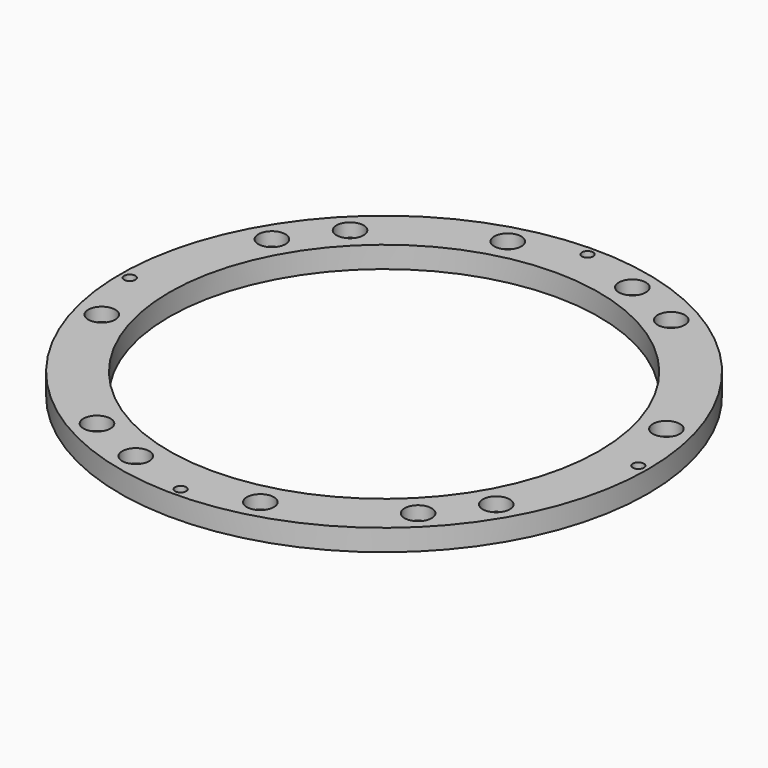
from build123d import *

# Parameters (mm, degrees)
F0_R     = 78
F0_R_2   = 2.375
F0_R_3   = 1.65
F0_R_4   = 63.5
F1_DEPTH = 6.35
F2_R     = 4
F3_DEPTH = 4


# Not quite as in the source:
# - a length typed as a fraction of an inch, garbled in the dataset ("3 / 203.2 mm" for 3/8 in), is restored


with BuildPart() as f1:
    # F0 (on Top) → F1 (new body)
    with BuildSketch(Plane.XY):
        Circle(F0_R)
        with Locations((-35.5625, -61.5960568442)):
            Circle(F0_R_2, mode=Mode.SUBTRACT)
        with Locations((-18.4085045829, -68.7014743948)):
            Circle(F0_R_2, mode=Mode.SUBTRACT)
        with Locations((-68.7014743948, -18.4085045829)):
            Circle(F0_R_2, mode=Mode.SUBTRACT)
        with Locations((0, -75.15)):
            Circle(F0_R_3, mode=Mode.SUBTRACT)
        with Locations((18.4085045829, -68.7014743948)):
            Circle(F0_R_2, mode=Mode.SUBTRACT)
        with Locations((50.2929698119, -50.2929698119)):
            Circle(F0_R_2, mode=Mode.SUBTRACT)
        with Locations((61.5960568442, -35.5625)):
            Circle(F0_R_2, mode=Mode.SUBTRACT)
        with Locations((-75.15, 0)):
            Circle(F0_R_3, mode=Mode.SUBTRACT)
        with Locations((-61.5960568442, 35.5625)):
            Circle(F0_R_2, mode=Mode.SUBTRACT)
        with Locations((-50.2929698119, 50.2929698119)):
            Circle(F0_R_2, mode=Mode.SUBTRACT)
        with Locations((-18.4085045829, 68.7014743948)):
            Circle(F0_R_2, mode=Mode.SUBTRACT)
        Circle(F0_R_4, mode=Mode.SUBTRACT)
        with Locations((75.15, 0)):
            Circle(F0_R_3, mode=Mode.SUBTRACT)
        with Locations((68.7014743948, 18.4085045829)):
            Circle(F0_R_2, mode=Mode.SUBTRACT)
        with Locations((0, 75.15)):
            Circle(F0_R_3, mode=Mode.SUBTRACT)
        with Locations((18.4085045829, 68.7014743948)):
            Circle(F0_R_2, mode=Mode.SUBTRACT)
        with Locations((35.5625, 61.5960568442)):
            Circle(F0_R_2, mode=Mode.SUBTRACT)
    extrude(amount=F1_DEPTH)

    # F2 (on face) → F3 (cut)
    with BuildSketch(Plane.XY.offset(6.35)):
        with Locations((68.7014743948, 18.4085045829)):
            Circle(F2_R)
        with Locations((35.5625, 61.5960568442)):
            Circle(F2_R)
        with Locations((18.4085045829, 68.7014743948)):
            Circle(F2_R)
        with Locations((-18.4085045829, 68.7014743948)):
            Circle(F2_R)
        with Locations((-50.2929698119, 50.2929698119)):
            Circle(F2_R)
        with Locations((-61.5960568442, 35.5625)):
            Circle(F2_R)
        with Locations((-68.7014743948, -18.4085045829)):
            Circle(F2_R)
        with Locations((-35.5625, -61.5960568442)):
            Circle(F2_R)
        with Locations((-18.4085045829, -68.7014743948)):
            Circle(F2_R)
        with Locations((18.4085045829, -68.7014743948)):
            Circle(F2_R)
        with Locations((50.2929698119, -50.2929698119)):
            Circle(F2_R)
        with Locations((61.5960568442, -35.5625)):
            Circle(F2_R)
    extrude(amount=-F3_DEPTH, mode=Mode.SUBTRACT)


solid = f1.part
